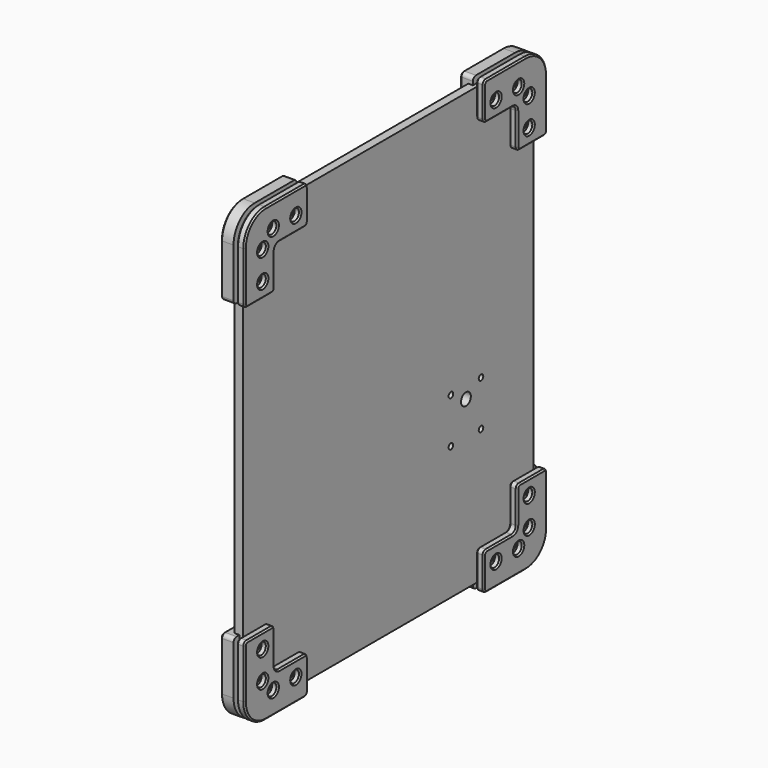
from build123d import *

# Parameters (mm, degrees)
F4_DEPTH        = 2.25
F5_R            = 1.5
F6_DEPTH        = 2.5
F8_DEPTH        = 4
F10_DEPTH       = 4
F12_DEPTH       = 2.6
F14_D           = 3.3
F14_CBORE_D     = 6
F14_CBORE_DEPTH = 3
F15_R           = 2
F16_SIZE        = 0.75
F17_SIZE        = 0.5
F19_D           = 3.3
F21_DEPTH       = 2.5
F22_R           = 2
F23_SIZE        = 0.5
F24_R           = 1.65
F25_DEPTH       = 0.2
F28_W           = 50
F28_H           = 36
F29_DEPTH       = 6
F30_R           = 3.25
F31_DEPTH       = 10.501
F32_R           = 1.5
F33_DEPTH       = 10.501


with BuildPart() as f4:
    # F3 (on Right) → F4 (new body, symmetric)
    with BuildSketch(Plane.YZ):
        with BuildLine():
            Line((86.5, 116), (-86.5, 116))
            ThreePointArc((-86.5, 116), (-93.5710678119, 113.0710678119), (-96.5, 106))
            Line((-96.5, 106), (-96.5, -106))
            ThreePointArc((-96.5, -106), (-93.5710678119, -113.0710678119), (-86.5, -116))
            Line((-86.5, -116), (86.5, -116))
            ThreePointArc((86.5, -116), (93.5710678119, -113.0710678119), (96.5, -106))
            Line((96.5, -106), (96.5, 106))
            ThreePointArc((96.5, 106), (93.5710678119, 113.0710678119), (86.5, 116))
        make_face()
    extrude(amount=F4_DEPTH, both=True)

    # F5 (on Right) → F6 (cut, symmetric)
    with BuildSketch(Plane.YZ):
        with Locations((-66.5, 108)):
            Circle(F5_R)
        with Locations((-81.5, 108)):
            Circle(F5_R)
        with Locations((-88.5, 101)):
            Circle(F5_R)
        with Locations((-88.5, 86)):
            Circle(F5_R)
        with Locations((66.5, 108)):
            Circle(F5_R)
        with Locations((81.5, 108)):
            Circle(F5_R)
        with Locations((88.5, 101)):
            Circle(F5_R)
        with Locations((88.5, 86)):
            Circle(F5_R)
        with Locations((88.5, -101)):
            Circle(F5_R)
        with Locations((88.5, -86)):
            Circle(F5_R)
        with Locations((81.5, -108)):
            Circle(F5_R)
        with Locations((66.5, -108)):
            Circle(F5_R)
        with Locations((-88.5, -86)):
            Circle(F5_R)
        with Locations((-88.5, -101)):
            Circle(F5_R)
        with Locations((-81.5, -108)):
            Circle(F5_R)
        with Locations((-66.5, -108)):
            Circle(F5_R)
    extrude(amount=F6_DEPTH, both=True, mode=Mode.SUBTRACT)

    # F30 (on face) → F31 (cut, through all)
    with BuildSketch(Plane.YZ.offset(2.25)):
        with Locations((51.5, -27.25)):
            Circle(F30_R)
    extrude(amount=-F31_DEPTH, mode=Mode.SUBTRACT)

    # F32 (on face) → F33 (cut, through all)
    with BuildSketch(Plane.YZ.offset(2.25)):
        with Locations((41.5, -45.25)):
            Circle(F32_R)
        with Locations((41.5, -21.25)):
            Circle(F32_R)
        with Locations((61.5, -21.25)):
            Circle(F32_R)
        with Locations((61.5, -45.25)):
            Circle(F32_R)
    extrude(amount=-F33_DEPTH, mode=Mode.SUBTRACT)


with BuildPart() as f8:
    # F7 (on face) → F8 (new body)
    with BuildSketch(Plane.YZ.offset(2.25)):
        with BuildLine():
            Line((-58.5, 100), (-58.5, 120))
            Line((-58.5, 120), (-86.5, 120))
            ThreePointArc((-86.5, 120), (-96.3994949366, 115.8994949366), (-100.5, 106))
            Line((-100.5, 106), (-100.5, 78))
            Line((-100.5, 78), (-80.5, 78))
            Line((-80.5, 78), (-80.5, 97))
            ThreePointArc((-80.5, 97), (-79.6213203436, 99.1213203436), (-77.5, 100))
            Line((-77.5, 100), (-58.5, 100))
        make_face()
    extrude(amount=F8_DEPTH)

    # F14 (through all)
    with Locations(Plane.YZ.offset(6.25)):
        with Locations((-88.5, 86), (-88.5, 101), (-81.5, 108), (-66.5, 108)):
            CounterBoreHole(F14_D / 2, F14_CBORE_D / 2, F14_CBORE_DEPTH)

    # F15
    f15_edges = [f8.edges().sort_by_distance(p)[0] for p in [
        (4.25, -58.5, 100),
        (4.25, -80.5, 78),
        (4.25, -58.5, 120),
        (4.25, -100.5, 78),
    ]]
    fillet(f15_edges, radius=F15_R)

    # F16
    f16_edges = [f8.edges().sort_by_distance(p)[0] for p in [
        (6.25, -58.5, 110),
        (6.25, -59.085786, 100.585786),
        (6.25, -59.085786, 119.414214),
        (6.25, -69, 100),
        (6.25, -73.5, 120),
        (6.25, -79.62132, 99.12132),
        (6.25, -96.399495, 115.899495),
        (6.25, -80.5, 88.5),
        (6.25, -100.5, 93),
        (6.25, -81.085786, 78.585786),
        (6.25, -99.914214, 78.585786),
        (6.25, -90.5, 78),
        (6.25, -91.5, 86),
        (6.25, -91.5, 101),
        (6.25, -84.5, 108),
        (6.25, -69.5, 108),
    ]]
    chamfer(f16_edges, length=F16_SIZE)

    # F17
    f17_edges = [f8.edges().sort_by_distance(p)[0] for p in [
        (2.25, -58.5, 110),
        (2.25, -59.085786, 100.585786),
        (2.25, -59.085786, 119.414214),
        (2.25, -69, 100),
        (2.25, -73.5, 120),
        (2.25, -79.62132, 99.12132),
        (2.25, -96.399495, 115.899495),
        (2.25, -80.5, 88.5),
        (2.25, -100.5, 93),
        (2.25, -81.085786, 78.585786),
        (2.25, -99.914214, 78.585786),
        (2.25, -90.5, 78),
        (2.25, -90.15, 86),
        (2.25, -90.15, 101),
        (2.25, -83.15, 108),
        (2.25, -68.15, 108),
    ]]
    chamfer(f17_edges, length=F17_SIZE)


with BuildPart() as f10:
    # F9 (on face) → F10 (new body)
    with BuildSketch(Plane(origin=(-2.25, 0, 0), x_dir=(0, -1, 0), z_dir=(-1, 0, 0))):
        with BuildLine():
            Line((58.5, 120), (58.5, 100))
            Line((58.5, 100), (77.5, 100))
            ThreePointArc((77.5, 100), (79.6213203436, 99.1213203436), (80.5, 97))
            Line((80.5, 97), (80.5, 78))
            Line((80.5, 78), (100.5, 78))
            Line((100.5, 78), (100.5, 106))
            ThreePointArc((100.5, 106), (96.3994949366, 115.8994949366), (86.5, 120))
            Line((86.5, 120), (58.5, 120))
        make_face()
    extrude(amount=F10_DEPTH)

    # F11 (on face) → F12 (join)
    with BuildSketch(Plane.YZ.offset(-2.25)):
        with BuildLine():
            Line((-100.5, 106), (-100.5, 78))
            Line((-100.5, 78), (-96.6, 78))
            Line((-96.6, 78), (-96.6, 106))
            ThreePointArc((-96.6, 106), (-93.64177849, 113.14177849), (-86.5, 116.1))
            Line((-86.5, 116.1), (-58.5, 116.1))
            Line((-58.5, 116.1), (-58.5, 120))
            Line((-58.5, 120), (-86.5, 120))
            ThreePointArc((-86.5, 120), (-96.3994949366, 115.8994949366), (-100.5, 106))
        make_face()
    extrude(amount=F12_DEPTH)

    # F19 (through all)
    with Locations(Plane.YZ.offset(-2.25)):
        with Locations((-88.5, 101), (-88.5, 86), (-81.5, 108), (-66.5, 108)):
            Hole(F19_D / 2)

    # F20 (on face) → F21 (cut)
    with BuildSketch(Plane(origin=(-6.25, 0, 0), x_dir=(0, -1, 0), z_dir=(-1, 0, 0))):
        Polygon((88.5, 89.4641016151), (85.5, 87.7320508076), (85.5, 84.2679491924), (88.5, 82.5358983849), (91.5, 84.2679491924), (91.5, 87.7320508076), align=None)
        Polygon((85.5, 102.7320508076), (85.5, 99.2679491924), (88.5, 97.5358983849), (91.5, 99.2679491924), (91.5, 102.7320508076), (88.5, 104.4641016151), align=None)
        Polygon((78.0358983849, 108), (79.7679491924, 105), (83.2320508076, 105), (84.9641016151, 108), (83.2320508076, 111), (79.7679491924, 111), align=None)
        Polygon((64.7679491924, 105), (68.2320508076, 105), (69.9641016151, 108), (68.2320508076, 111), (64.7679491924, 111), (63.0358983849, 108), align=None)
    extrude(amount=-F21_DEPTH, mode=Mode.SUBTRACT)

    # F22
    f22_edges = [f10.edges().sort_by_distance(p)[0] for p in [
        (-4.25, -58.5, 100),
        (-4.25, -80.5, 78),
        (-2.95, -100.5, 78),
        (-2.95, -58.5, 120),
    ]]
    fillet(f22_edges, radius=F22_R)

    # F23
    f23_edges = [f10.edges().sort_by_distance(p)[0] for p in [
        (-6.25, -58.5, 110),
        (-6.25, -59.085786, 119.414214),
        (-6.25, -59.085786, 100.585786),
        (-6.25, -73.5, 120),
        (-6.25, -69, 100),
        (-6.25, -96.399495, 115.899495),
        (-6.25, -79.62132, 99.12132),
        (-6.25, -100.5, 93),
        (-6.25, -80.5, 88.5),
        (-6.25, -99.914214, 78.585786),
        (-6.25, -81.085786, 78.585786),
        (-6.25, -90.5, 78),
        (-6.25, -90, 88.598076),
        (-6.25, -87, 88.598076),
        (-6.25, -85.5, 86),
        (-6.25, -87, 83.401924),
        (-6.25, -90, 83.401924),
        (-6.25, -91.5, 86),
        (-6.25, -63.901924, 106.5),
        (-6.25, -66.5, 105),
        (-6.25, -69.098076, 106.5),
        (-6.25, -69.098076, 109.5),
        (-6.25, -66.5, 111),
        (-6.25, -63.901924, 109.5),
        (-6.25, -85.5, 101),
        (-6.25, -87, 98.401924),
        (-6.25, -90, 98.401924),
        (-6.25, -91.5, 101),
        (-6.25, -90, 103.598076),
        (-6.25, -87, 103.598076),
        (-6.25, -78.901924, 106.5),
        (-6.25, -81.5, 105),
        (-6.25, -84.098076, 106.5),
        (-6.25, -84.098076, 109.5),
        (-6.25, -81.5, 111),
        (-6.25, -78.901924, 109.5),
    ]]
    chamfer(f23_edges, length=F23_SIZE)

    # F24 (on face) → F25 (join)
    with BuildSketch(Plane(origin=(-3.75, 0, 0), x_dir=(0, -1, 0), z_dir=(-1, 0, 0))):
        with Locations((88.5, 86)):
            Circle(F24_R)
        with Locations((88.5, 101)):
            Circle(F24_R)
        with Locations((81.5, 108)):
            Circle(F24_R)
        with Locations((66.5, 108)):
            Circle(F24_R)
    extrude(amount=-F25_DEPTH)


with BuildPart() as f26_1:
    # F26: instance of F8
    add(f8.part.mirror(Plane.XZ))


with BuildPart() as f26_2:
    # F26: instance of F10
    add(f10.part.mirror(Plane.XZ))


with BuildPart() as f27_1:
    # F27: instance of F8
    add(f8.part.mirror(Plane.XY))


with BuildPart() as f27_2:
    # F27: instance of F10
    add(f10.part.mirror(Plane.XY))


with BuildPart() as f27_3:
    # F27: instance of F26_1
    add(f26_1.part.mirror(Plane.XY))


with BuildPart() as f27_4:
    # F27: instance of F26_2
    add(f26_2.part.mirror(Plane.XY))


with BuildPart() as f29:
    # F28 (on face) → F29 (new body)
    with BuildSketch(Plane(origin=(-2.25, 0, 0), x_dir=(0, -1, 0), z_dir=(-1, 0, 0))):
        with Locations((30, -42)):
            Rectangle(F28_W, F28_H)
    extrude(amount=F29_DEPTH)


solid = Compound([f4.part, f8.part, f10.part, f26_1.part, f26_2.part, f27_1.part, f27_2.part, f27_3.part, f27_4.part, f29.part])
